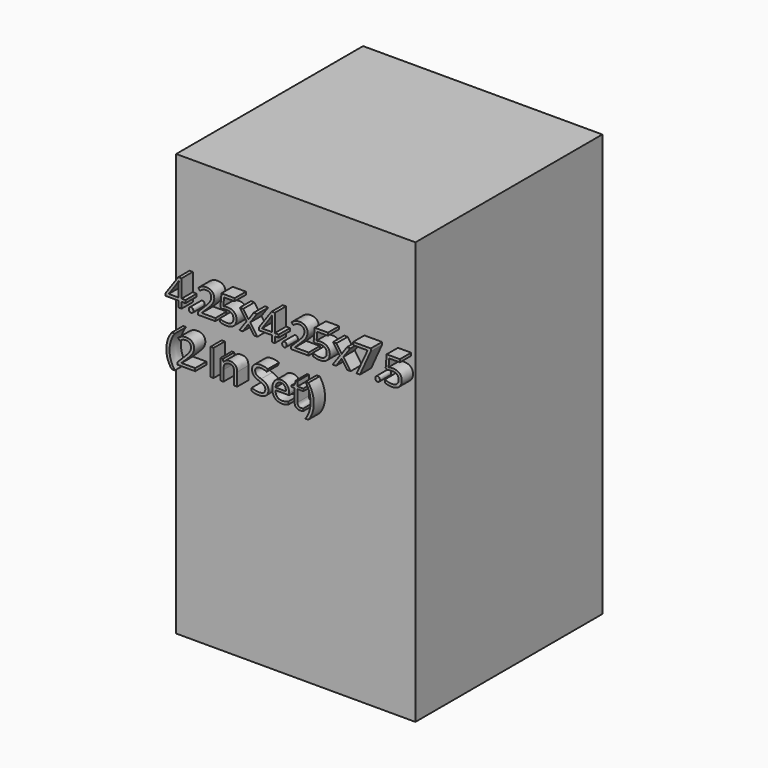
from build123d import *

# Parameters (mm, degrees)
F0_W         = 107.95
F0_H         = 190.5
F1_DEPTH     = 105.41
F2_TEXT_SIZE = 16.7958379929
F3_DEPTH     = 6.35


# Not quite as in the source:
# - Text() gives the source's letters only with a copy of the font that has no kerning and outlines rounded to 1/6400 em; it was checked with that copy


with BuildPart() as f1:
    # F0 (on Front) → F1 (new body)
    with BuildSketch(Plane.XZ):
        with Locations((53.975, 95.25)):
            Rectangle(F0_W, F0_H)
    extrude(amount=F1_DEPTH)

    # F2 (on face) → F3 (join)
    with BuildSketch(Plane.XZ.offset(105.41)):
        with Locations((0, 134.0477132922)):
            Text('4.25x4.25x7.5', F2_TEXT_SIZE, font='Open Sans', text_align=(TextAlign.LEFT, TextAlign.BOTTOM))
        with Locations((0, 111.2053736218)):
            Text('(2 In Set)', F2_TEXT_SIZE, font='Open Sans', text_align=(TextAlign.LEFT, TextAlign.BOTTOM))
    extrude(amount=F3_DEPTH)


solid = f1.part
